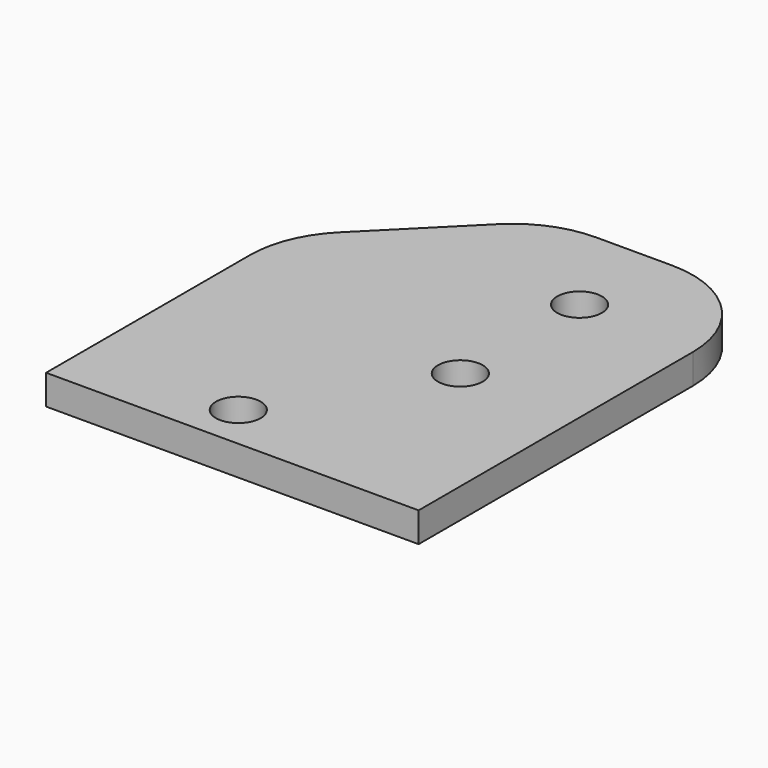
from build123d import *

# Parameters (mm, degrees)
F0_W        = 25
F0_H        = 30
F1_DEPTH    = 2
F2_R        = 1.5
F3_DEPTH    = 2.001
F4_W        = 1
F4_H        = 6.1
F5_DEPTH    = 0.9
F6_T1_DEPTH = 53.4336597593
F7_R        = 7


# Not quite as in the source:
# - a fillet or chamfer that OpenCascade refuses, or shapes differently, is made with other operations: its cross-section is extruded or revolved along the edge and cut away or added


with BuildPart() as f1:
    # F0 (on Top) → F1 (new body)
    with BuildSketch(Plane.XY):
        Rectangle(F0_W, F0_H)
    extrude(amount=F1_DEPTH)

    # F2 (on face) → F3 (cut, through all)
    with BuildSketch(Plane.XY.offset(2)):
        with Locations((-2, -12)):
            Circle(F2_R)
        with Locations((4.5, -1.5)):
            Circle(F2_R)
        with Locations((4.5, 8.5)):
            Circle(F2_R)
    extrude(amount=-F3_DEPTH, mode=Mode.SUBTRACT)

    # F4 (on face) → F5 (cut)
    with BuildSketch(Plane(origin=(0, 0, 0), x_dir=(1, 0, 0), z_dir=(0, 0, -1))):
        with Locations((11.6, -3.051)):
            Rectangle(F4_W, F4_H)
        with Locations((9.6, -3.051)):
            Rectangle(F4_W, F4_H)
        with Locations((7.6, -3.051)):
            Rectangle(F4_W, F4_H)
        with Locations((5.6, -3.051)):
            Rectangle(F4_W, F4_H)
        with Locations((3.6, -3.051)):
            Rectangle(F4_W, F4_H)
        with Locations((1.6, -3.051)):
            Rectangle(F4_W, F4_H)
        with Locations((-0.4, -3.051)):
            Rectangle(F4_W, F4_H)
        with Locations((-2.4, -3.051)):
            Rectangle(F4_W, F4_H)
        with Locations((-4.4, -3.051)):
            Rectangle(F4_W, F4_H)
        with Locations((-6.4, -3.051)):
            Rectangle(F4_W, F4_H)
        with Locations((-8.4, -3.051)):
            Rectangle(F4_W, F4_H)
        with Locations((-10.4, -3.051)):
            Rectangle(F4_W, F4_H)
        with Locations((-12.4, -3.051)):
            Rectangle(F4_W, F4_H)
    extrude(amount=-F5_DEPTH, mode=Mode.SUBTRACT)

    # F6: chamfer of 10 on 1 edges, made by hand

    # F6_s2 → F6_t1 (cut)
    with BuildSketch(Plane.XY.offset(-25.7168298797)):
        Polygon((-12.5, 5), (-2.5, 15), (-12.5, 15), align=None)
    extrude(amount=F6_T1_DEPTH, mode=Mode.SUBTRACT)

    # F7
    f7_edges = [f1.edges().sort_by_distance(p)[0] for p in [
        (-12.5, 5, 1.45),
        (-2.5, 15, 1),
        (12.5, 15, 1),
    ]]
    fillet(f7_edges, radius=F7_R)


solid = f1.part
